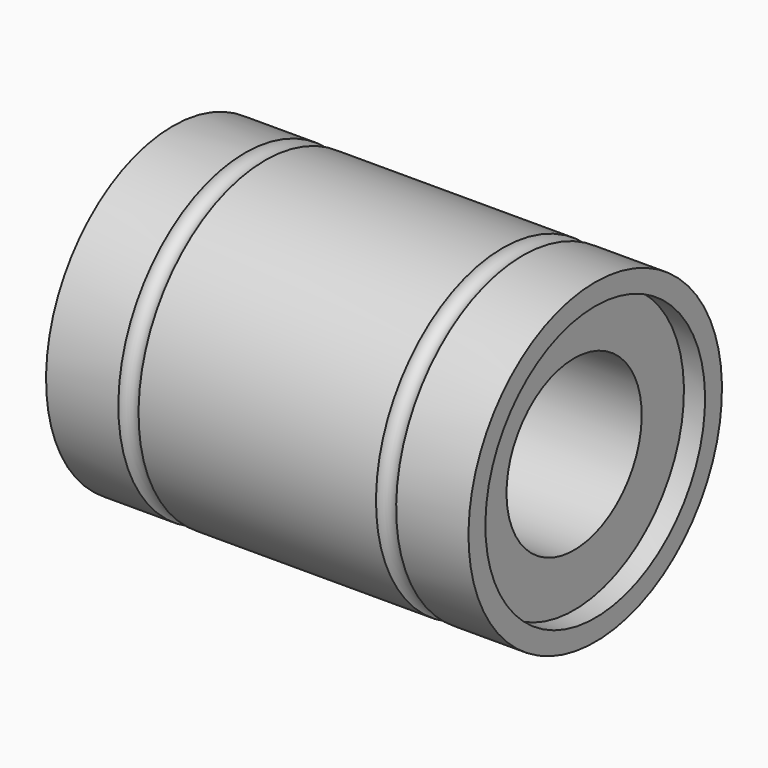
from build123d import *

# Parameters (mm, degrees)
F2_DEPTH = 25


# Not quite as in the source:
# - a feature names something its author has since deleted; it is built from what else it names


with BuildPart() as f1:
    # F0 (on Front) → F1 (revolve)
    with BuildSketch(Plane.XZ):
        with BuildLine():
            Line((0, 9.9311807901), (0, 10.9311807901))
            Line((0, 10.9311807901), (-3.4236455734, 10.9311807901))
            ThreePointArc((-3.4236455734, 10.9311807901), (-3.9013040029, 10.5789726191), (-4.3789624324, 10.9311807901))
            Line((-4.3789624324, 10.9311807901), (-15.6210375676, 10.9311807901))
            ThreePointArc((-15.6210375676, 10.9311807901), (-16.0986959971, 10.5789726191), (-16.5763544266, 10.9311807901))
            Line((-16.5763544266, 10.9311807901), (-20, 10.9311807901))
            Line((-20, 10.9311807901), (-20, 9.9311807901))
            Line((-20, 9.9311807901), (-19, 9.9311807901))
            Line((-19, 9.9311807901), (-19, 7.4311807901))
            Line((-19, 7.4311807901), (-18.118519783, 7.4311807901))
            Line((-18.118519783, 7.4311807901), (-18.118519783, 3.4311807901))
            Line((-18.118519783, 3.4311807901), (-1.881480217, 3.4311807901))
            Line((-1.881480217, 3.4311807901), (-1.881480217, 7.4311807901))
            Line((-1.881480217, 7.4311807901), (-1, 7.4311807901))
            Line((-1, 7.4311807901), (-1, 9.9311807901))
            Line((-1, 9.9311807901), (0, 9.9311807901))
        make_face()
    revolve(axis=Axis((-10, 0, 3.4311807901), (-1, 0, 0)))

    # F2 (cut): a face of the model
    f2_faces = [f1.faces().sort_by_distance(p)[0] for p in [
        (-18.118519783, 0, 3.4311807901),
    ]]
    extrude(f2_faces, amount=-F2_DEPTH, mode=Mode.SUBTRACT)


solid = f1.part
